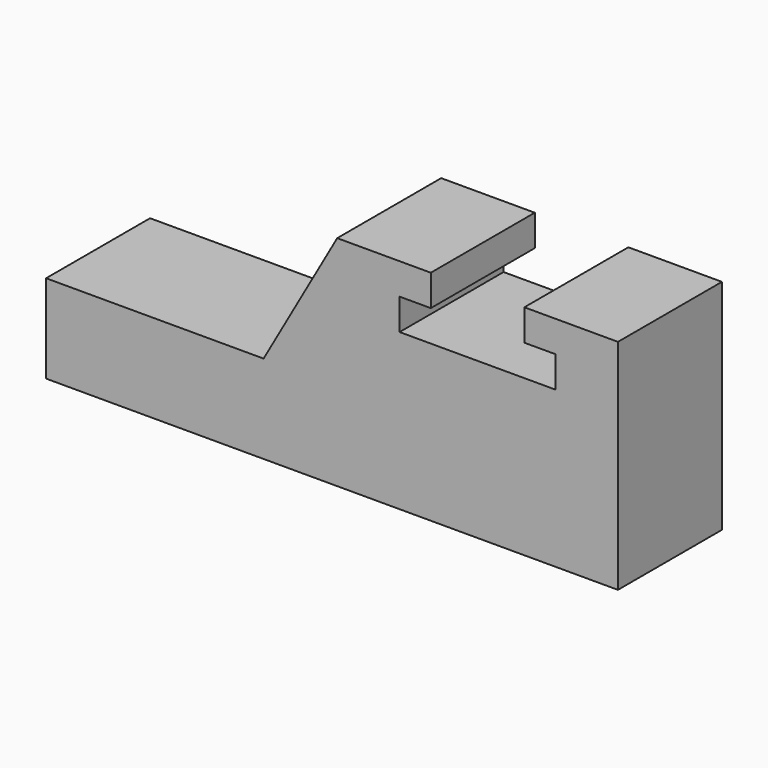
from build123d import *

# Parameters (mm, degrees)
F2_DEPTH = 635
F3_DEPTH = 635


with BuildPart() as f2:
    # F1 (on face) → F2 (new body)
    with BuildSketch(Plane.XZ):
        Polygon((0, -431.8), (0, 0), (-1524, 0), (-1731.2896251678, 0), (-2540, 0), (-2794, 0), (-2794, -431.8), align=None)
        Polygon((-1524, 0), (0, 0), (0, 635), (-457.2, 635), (-457.2, 482.6), (-304.8, 482.6), (-304.8, 330.2), (-1066.8, 330.2), (-1066.8, 482.6), (-914.4, 482.6), (-914.4, 635), (-1371.6, 635), (-1731.2896251678, 0), align=None)
    extrude(amount=F2_DEPTH)

    # F0 (on Front) → F3 (join)
    with BuildSketch(Plane.XZ):
        Polygon((-1731.2896251678, 0), (0, 0), (0, 635), (-457.2, 635), (-457.2, 482.6), (-304.8, 482.6), (-304.8, 330.2), (-1066.8, 330.2), (-1066.8, 482.6), (-914.4, 482.6), (-914.4, 635), (-1371.6, 635), align=None)
    extrude(amount=F3_DEPTH)


solid = f2.part
